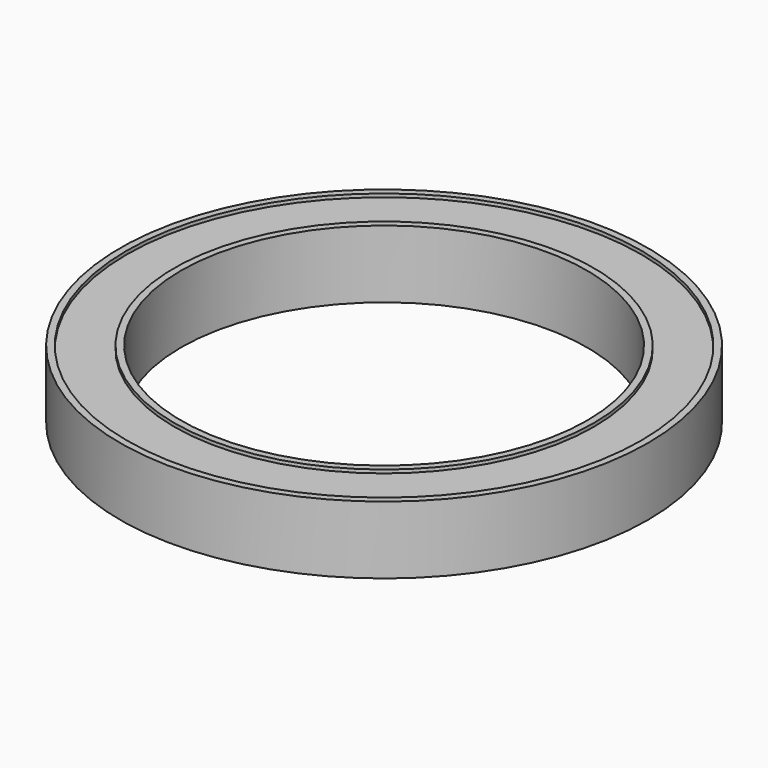
from build123d import *

# Parameters (mm, degrees)
F0_R     = 39
F0_R_2   = 30
F1_DEPTH = 5
F2_R     = 38
F2_R_2   = 31
F3_DEPTH = 0.5


# Not quite as in the source:
# - a pattern or mirror of a feature is missing from the dataset's text; its kind, count and spacing are read off the source's solid


with BuildPart() as f1:
    # F0 (on Top) → F1 (new body, symmetric)
    with BuildSketch(Plane.XY):
        Circle(F0_R)
        Circle(F0_R_2, mode=Mode.SUBTRACT)
    extrude(amount=F1_DEPTH, both=True)

    # F2 (on face) → F3 (cut)
    with BuildSketch(Plane.XY.offset(5)):
        Circle(F2_R)
        Circle(F2_R_2, mode=Mode.SUBTRACT)
    f3 = extrude(amount=-F3_DEPTH, mode=Mode.SUBTRACT)

    # F3_copies: F3 across plane
    add(f3.mirror(Plane(origin=(0, 0, 0), x_dir=(-1, 0, 0), z_dir=(0, 0, -1))), mode=Mode.SUBTRACT)


solid = f1.part
